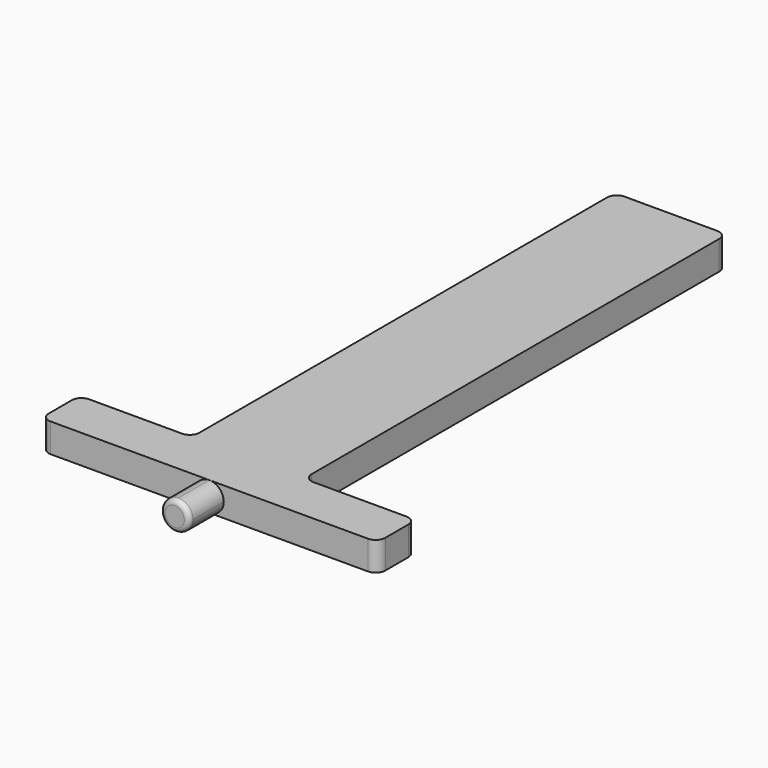
from build123d import *

# Parameters (mm, degrees)
F4_DEPTH = 3
F6_DEPTH = 4.5


# Not quite as in the source:
# - a fillet or chamfer that OpenCascade refuses, or shapes differently, is made with other operations: its cross-section is extruded or revolved along the edge and cut away or added


with BuildPart() as f4:
    # F3 (on Top) → F4 (new body)
    with BuildSketch(Plane.XY):
        with BuildLine():
            ThreePointArc((0, 1), (0.2928932188, 0.2928932188), (1, 0))
            Line((1, 0), (34, 0))
            ThreePointArc((34, 0), (34.7071067812, 0.2928932188), (35, 1))
            Line((35, 1), (35, 4))
            ThreePointArc((35, 4), (34.7071067812, 4.7071067812), (34, 5))
            Line((34, 5), (24.3333333333, 5))
            ThreePointArc((24.3333333333, 5), (23.6262265521, 5.2928932188), (23.3333333333, 6))
            Line((23.3333333333, 6), (23.3333333333, 59))
            ThreePointArc((23.3333333333, 59), (23.0404401145, 59.7071067812), (22.3333333333, 60))
            Line((22.3333333333, 60), (12.6666666667, 60))
            ThreePointArc((12.6666666667, 60), (11.9595598855, 59.7071067812), (11.6666666667, 59))
            Line((11.6666666667, 59), (11.6666666667, 6))
            ThreePointArc((11.6666666667, 6), (11.3737734479, 5.2928932188), (10.6666666667, 5))
            Line((10.6666666667, 5), (1, 5))
            ThreePointArc((1, 5), (0.2928932188, 4.7071067812), (0, 4))
            Line((0, 4), (0, 1))
        make_face()
    extrude(amount=F4_DEPTH)

    # F5 (on face) → F6 (join)
    with BuildSketch(Plane.XZ):
        with BuildLine():
            ThreePointArc((17.5, 0), (18.5606601718, 0.4393398282), (19, 1.5))
            ThreePointArc((19, 1.5), (18.5606601718, 2.5606601718), (17.5, 3))
            ThreePointArc((17.5, 3), (16, 1.5), (17.5, 0))
        make_face()
    extrude(amount=F6_DEPTH)

    # F7: fillet of radius 0.5 on 1 edges, made by hand

    # F7_s1 → F7_t2 (revolve, cut)
    with BuildSketch(Plane.YZ.offset(17.5)):
        with BuildLine():
            ThreePointArc((-4, 0), (-4.3535533906, 0.1464466094), (-4.5, 0.5))
            Line((-4.5, 0.5), (-4.5, 0))
            Line((-4.5, 0), (-4, 0))
        make_face()
    revolve(axis=Axis((17.5, -4.5, 1.5), (0, 1, 0)), mode=Mode.SUBTRACT)


solid = f4.part
